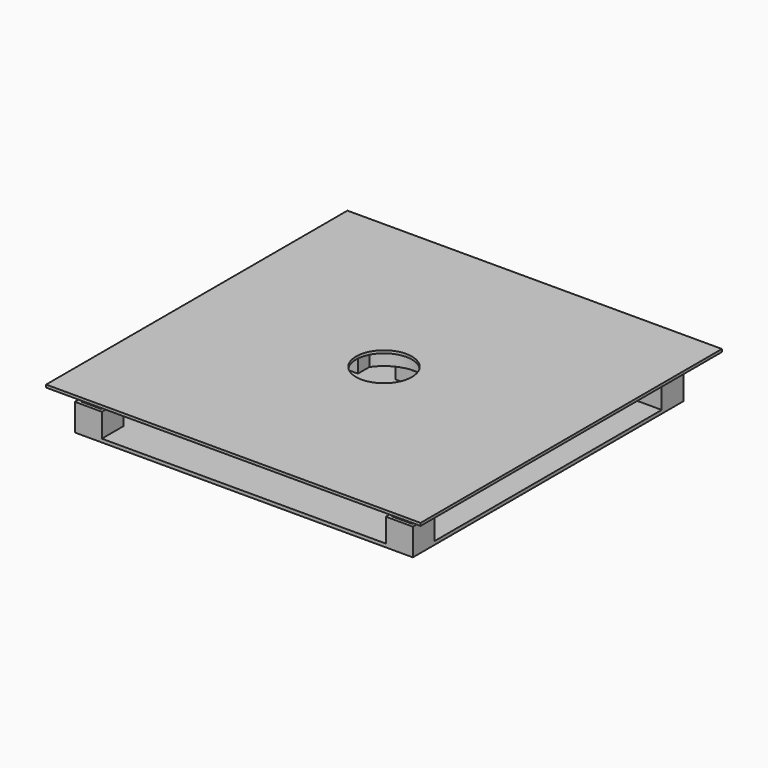
from build123d import *

# Parameters (mm, degrees)
F0_W          = 50
F0_H          = 50
F1_DEPTH      = 0.5
F2_W          = 4
F2_H          = 4
F2_W_2        = 3
F2_H_2        = 3
F3_DEPTH      = 3.5
F2_W_3        = 1.9
F2_H_3        = 1.9
F4_DEPTH      = 6
F5_W          = 55.382803781
F5_H          = 55.7085196488
F5_W_2        = 1.9
F5_H_2        = 1.9
F6_DEPTH      = 0.4
F7_R          = 4.125
F8_DEPTH      = 25
F9_R          = 6.25
F10_DEPTH     = 2.5
F11_W         = 7.5
F11_H         = 3.75
F11_H_2       = 7.5
F12_DEPTH     = 2
F13_W         = 4.95
F13_H         = 0.875
F14_DEPTH     = 1
F15_R         = 1.5
F16_W         = 15
F16_H         = 2.25
F17_DEPTH     = 2.5
F19_DEPTH     = 1
F20_W         = 5
F20_H         = 5
F21_DEPTH     = 1.05
F22_T4_DEPTH  = 11.4471090443
F22_T9_DEPTH  = 11.4471090443
F22_T14_DEPTH = 11.4471090443
F22_T19_DEPTH = 11.4471090443


# Not quite as in the source:
# - a fillet or chamfer that OpenCascade refuses, or shapes differently, is made with other operations: its cross-section is extruded or revolved along the edge and cut away or added
# - a feature names something its author has since deleted; it is built from what else it names


with BuildPart() as f1:
    # F0 (on Top) → F1 (new body)
    with BuildSketch(Plane.XY):
        with Locations((25, 25)):
            Rectangle(F0_W, F0_H)
    extrude(amount=F1_DEPTH)

    # F2 (on face) → F3 (join)
    with BuildSketch(Plane.XY.offset(0.5)):
        with Locations((48, 48)):
            Rectangle(F2_W, F2_H)
        with Locations((48, 48)):
            Rectangle(F2_W_2, F2_H_2, mode=Mode.SUBTRACT)
        with Locations((2, 48)):
            Rectangle(F2_W, F2_H)
        with Locations((2, 48)):
            Rectangle(F2_W_2, F2_H_2, mode=Mode.SUBTRACT)
        with Locations((2, 2)):
            Rectangle(F2_W, F2_H)
        with Locations((2, 2)):
            Rectangle(F2_W_2, F2_H_2, mode=Mode.SUBTRACT)
        with Locations((48, 2)):
            Rectangle(F2_W, F2_H)
        with Locations((48, 2)):
            Rectangle(F2_W_2, F2_H_2, mode=Mode.SUBTRACT)
    extrude(amount=F3_DEPTH)

    # F11 (on face) → F12 (join)
    with BuildSketch(Plane.XY.offset(0.5)):
        with Locations((13.5, 26.875)):
            Rectangle(F11_W, F11_H)
        with Locations((13.5, 23.125)):
            Rectangle(F11_W, F11_H)
        with Locations((25, 13.5)):
            Rectangle(F11_W, F11_H_2)
        with Locations((36.5, 25)):
            Rectangle(F11_W, F11_H_2)
        with Locations((25, 36.5)):
            Rectangle(F11_W, F11_H_2)
    extrude(amount=F12_DEPTH)

    # F13 (on face) → F14 (join)
    with BuildSketch(Plane.XY.offset(2.5)):
        Polygon((15.975, 22.125), (15.975, 21.25), (17.25, 21.25), (17.25, 28.75), (15.975, 28.75), align=None)
        with Locations((13.5, 21.6875)):
            Rectangle(F13_W, F13_H)
        Polygon((9.75, 21.25), (11.025, 21.25), (11.025, 22.125), (11.025, 28.75), (9.75, 28.75), align=None)
    extrude(amount=F14_DEPTH)

    # F15
    f15_edges = [f1.edges().sort_by_distance(p)[0] for p in [
        (9.75, 28.75, 2),
        (17.25, 28.75, 2),
        (17.25, 21.25, 2),
        (9.75, 21.25, 2),
    ]]
    fillet(f15_edges, radius=F15_R)


with BuildPart() as f4:
    # F2 (on face) → F4 (new body)
    with BuildSketch(Plane.XY.offset(0.5)):
        with Locations((2, 48)):
            Rectangle(F2_W_3, F2_H_3)
    extrude(amount=F4_DEPTH)



with BuildPart() as f4b:
    # F2 (on face) → F4, piece 2 (new body)
    with BuildSketch(Plane.XY.offset(0.5)):
        with Locations((48, 48)):
            Rectangle(F2_W_3, F2_H_3)
    extrude(amount=F4_DEPTH)


with BuildPart() as f4c:
    # F2 (on face) → F4, piece 3 (new body)
    with BuildSketch(Plane.XY.offset(0.5)):
        with Locations((48, 2)):
            Rectangle(F2_W_3, F2_H_3)
    extrude(amount=F4_DEPTH)


with BuildPart() as f4d:
    # F2 (on face) → F4, piece 4 (new body)
    with BuildSketch(Plane.XY.offset(0.5)):
        with Locations((2, 2)):
            Rectangle(F2_W_3, F2_H_3)
    extrude(amount=F4_DEPTH)


with BuildPart() as f4_1:
    add(f4.part)

    add(f4b.part)  # F6 merges F4b

    add(f4c.part)  # F6 merges F4c

    add(f4d.part)  # F6 merges F4d
    # F5 (on face) → F6 (join)
    with BuildSketch(Plane.XY.offset(6.5)):
        with Locations((25.4082191968, 25.3989326302)):
            Rectangle(F5_W, F5_H)
        with Locations((48, 48)):
            Rectangle(F5_W_2, F5_H_2, mode=Mode.SUBTRACT)
    extrude(amount=-F6_DEPTH)

    # F7 (on face) → F8 (cut)
    with BuildSketch(Plane.XY.offset(6.5)):
        with Locations((25.4082191968, 25.3989326302)):
            Circle(F7_R)
    extrude(amount=-F8_DEPTH, mode=Mode.SUBTRACT)

    # F9 (on face) → F10 (join)
    with BuildSketch(Plane(origin=(0, 0, 6.1), x_dir=(1, 0, 0), z_dir=(0, 0, -1))):
        with Locations((25.4082191968, -25.3989326302)):
            Circle(F9_R)
        with BuildLine():
            ThreePointArc((30.1582191968, -22.158562281), (30.9025344408, -23.7033501344), (31.1582191968, -25.3989326302))
            ThreePointArc((31.1582191968, -25.3989326302), (30.9025344408, -27.094515126), (30.1582191968, -28.6393029794))
            ThreePointArc((30.1582191968, -28.6393029794), (25.4082191968, -31.1489326302), (20.6582191968, -28.6393029794))
            ThreePointArc((20.6582191968, -28.6393029794), (19.6582191968, -25.3989326302), (20.6582191968, -22.158562281))
            ThreePointArc((20.6582191968, -22.158562281), (25.4082191968, -19.6489326302), (30.1582191968, -22.158562281))
        make_face(mode=Mode.SUBTRACT)
        with BuildLine():
            ThreePointArc((30.1582191968, -28.6393029794), (30.9025344408, -27.094515126), (31.1582191968, -25.3989326302))
            ThreePointArc((31.1582191968, -25.3989326302), (30.9025344408, -23.7033501344), (30.1582191968, -22.158562281))
            Line((30.1582191968, -22.158562281), (30.1582191968, -28.6393029794))
        make_face()
        with BuildLine():
            Line((20.6582191968, -28.6393029794), (20.6582191968, -22.158562281))
            ThreePointArc((20.6582191968, -22.158562281), (19.6582191968, -25.3989326302), (20.6582191968, -28.6393029794))
        make_face()
    extrude(amount=F10_DEPTH)

    # F16 (on face) → F17 (cut, through all)
    with BuildSketch(Plane(origin=(0, 0, 3.6), x_dir=(1, 0, 0), z_dir=(0, 0, -1))):
        with Locations((25.4082191968, -25.3989326302)):
            Rectangle(F16_W, F16_H)
    extrude(amount=-F17_DEPTH, mode=Mode.SUBTRACT)


with BuildPart() as f19:
    # F18 (on Top) → F19 (new body)
    with BuildSketch(Plane.XY):
        with BuildLine():
            ThreePointArc((29.6416427523, 25.0239326302), (29.6540730633, 25.2112495339), (29.6582191968, 25.3989326302))
            ThreePointArc((29.6582191968, 25.3989326302), (29.6540730633, 25.5866157265), (29.6416427523, 25.7739326302))
            Line((29.6416427523, 25.7739326302), (25.4082191968, 25.7739326302))
            Line((25.4082191968, 25.7739326302), (21.1747956414, 25.7739326302))
            ThreePointArc((21.1747956414, 25.7739326302), (21.1582191968, 25.3989326302), (21.1747956414, 25.0239326302))
            Line((21.1747956414, 25.0239326302), (25.4082191968, 25.0239326302))
            Line((25.4082191968, 25.0239326302), (29.6416427523, 25.0239326302))
        make_face()
        with BuildLine():
            ThreePointArc((29.6416427523, 25.7739326302), (29.6540730633, 25.5866157265), (29.6582191968, 25.3989326302))
            ThreePointArc((29.6582191968, 25.3989326302), (29.6540730633, 25.2112495339), (29.6416427523, 25.0239326302))
            Line((29.6416427523, 25.0239326302), (32.2061355105, 25.0239326302))
            Line((32.2061355105, 25.0239326302), (32.2061355105, 25.3989326302))
            Line((32.2061355105, 25.3989326302), (32.2061355105, 25.7739326302))
            Line((32.2061355105, 25.7739326302), (29.6416427523, 25.7739326302))
        make_face()
        with BuildLine():
            Line((25.4082191968, 25.7739326302), (29.6416427523, 25.7739326302))
            ThreePointArc((29.6416427523, 25.7739326302), (25.4082191968, 29.6489326302), (21.1747956414, 25.7739326302))
            Line((21.1747956414, 25.7739326302), (25.4082191968, 25.7739326302))
        make_face()
        with BuildLine():
            ThreePointArc((21.1747956414, 25.0239326302), (25.4082191968, 21.1489326302), (29.6416427523, 25.0239326302))
            Line((29.6416427523, 25.0239326302), (25.4082191968, 25.0239326302))
            Line((25.4082191968, 25.0239326302), (21.1747956414, 25.0239326302))
        make_face()
        with BuildLine():
            ThreePointArc((21.1747956414, 25.0239326302), (21.1582191968, 25.3989326302), (21.1747956414, 25.7739326302))
            Line((21.1747956414, 25.7739326302), (18.6103028832, 25.7739326302))
            Line((18.6103028832, 25.7739326302), (18.6103028832, 25.3989326302))
            Line((18.6103028832, 25.3989326302), (18.6103028832, 25.0239326302))
            Line((18.6103028832, 25.0239326302), (21.1747956414, 25.0239326302))
        make_face()
    extrude(amount=-F19_DEPTH)

    # F20 (on face) → F21 (join)
    with BuildSketch(Plane(origin=(0, 0, -1), x_dir=(1, 0, 0), z_dir=(0, 0, -1))):
        with Locations((25.4082191968, -25.3989326302)):
            Rectangle(F20_W, F20_H)
    extrude(amount=F21_DEPTH)

    # F22: chamfer of 1 x 1.25 on 4 edges, made by hand


with BuildPart() as f22_tool2:
    # F22_s3 → F22_t4 (new body)
    with BuildSketch(Plane.XZ.offset(-31.1224871524)):
        Polygon((27.9082191968, -0.8), (26.9082191968, -2.05), (27.9082191968, -2.05), align=None)
    extrude(amount=F22_T4_DEPTH)

    split(bisect_by=Plane.XY.offset(-1), keep=Keep.BOTTOM)


with BuildPart() as f19_1:
    add(f19.part)

    # F22_t1: cut F22_tool2
    add(f22_tool2.part, mode=Mode.SUBTRACT)


with BuildPart() as f22_tool7:
    # F22_s8 → F22_t9 (new body)
    with BuildSketch(Plane.YZ.offset(31.131773719)):
        Polygon((22.8989326302, -0.8), (23.8989326302, -2.05), (22.8989326302, -2.05), align=None)
    extrude(amount=-F22_T9_DEPTH)

    split(bisect_by=Plane.XY.offset(-1), keep=Keep.BOTTOM)


with BuildPart() as f19_2:
    add(f19_1.part)

    # F22_t6: cut F22_tool7
    add(f22_tool7.part, mode=Mode.SUBTRACT)


with BuildPart() as f22_tool12:
    # F22_s13 → F22_t14 (new body)
    with BuildSketch(Plane.XZ.offset(-19.675378108)):
        Polygon((22.9082191968, -0.8), (23.9082191968, -2.05), (22.9082191968, -2.05), align=None)
    extrude(amount=-F22_T14_DEPTH)

    split(bisect_by=Plane.XY.offset(-1), keep=Keep.BOTTOM)


with BuildPart() as f19_3:
    add(f19_2.part)

    # F22_t11: cut F22_tool12
    add(f22_tool12.part, mode=Mode.SUBTRACT)


with BuildPart() as f22_tool17:
    # F22_s18 → F22_t19 (new body)
    with BuildSketch(Plane.YZ.offset(19.6846646747)):
        Polygon((27.8989326302, -0.8), (26.8989326302, -2.05), (27.8989326302, -2.05), align=None)
    extrude(amount=F22_T19_DEPTH)

    split(bisect_by=Plane.XY.offset(-1), keep=Keep.BOTTOM)


with BuildPart() as f19_4:
    add(f19_3.part)

    # F22_t16: cut F22_tool17
    add(f22_tool17.part, mode=Mode.SUBTRACT)


solid = Compound([f1.part, f4_1.part, f19_4.part])
